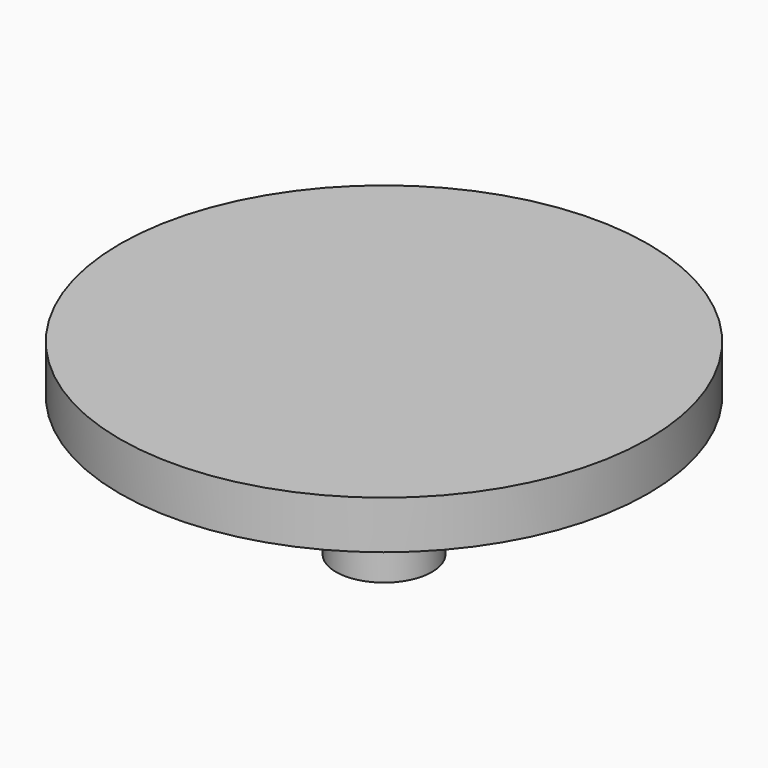
from build123d import *

# Parameters (mm, degrees)
F0_R         = 11
F1_DEPTH     = 2
F2_R         = 2
F3_DEPTH     = 5.8
F4_TEXT_SIZE = 7.3223669056
F5_DEPTH     = 1


# Not quite as in the source:
# - Text() gives the source's letters only with a copy of the font that has no kerning and outlines rounded to 1/6400 em; it was checked with that copy


with BuildPart() as f1:
    # F0 (on Top) → F1 (new body)
    with BuildSketch(Plane.XY):
        Circle(F0_R)
    extrude(amount=F1_DEPTH)

    # F2 (on face) → F3 (join)
    with BuildSketch(Plane(origin=(0, 0, 0), x_dir=(1, 0, 0), z_dir=(0, 0, -1))):
        Circle(F2_R)
    extrude(amount=F3_DEPTH)

    # F4 (on face) → F5 (join)
    with BuildSketch(Plane.XY.offset(2)):
        with Locations((-9.4539879356, -2.6197799016)):
            Text('Lewis', F4_TEXT_SIZE, font='Open Sans', text_align=(TextAlign.LEFT, TextAlign.BOTTOM))
    extrude(amount=-F5_DEPTH)


solid = f1.part
